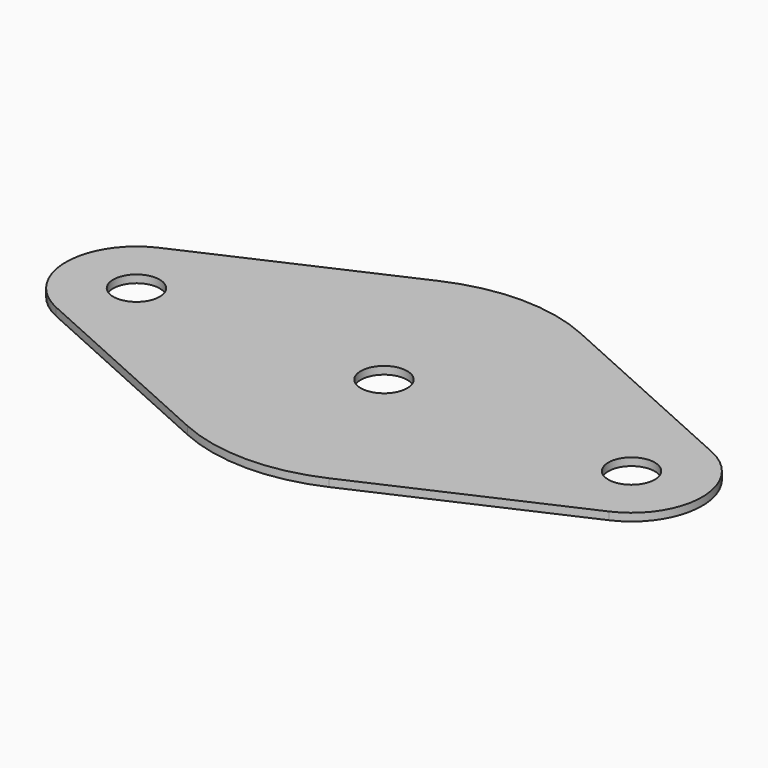
from build123d import *

# Parameters (mm, degrees)
F0_R     = 13.9065
F0_R_2   = 9.525
F1_DEPTH = 3.175


# Not quite as in the source:
# - a length typed as a fraction of an inch, garbled in the dataset ("3 / 203.2 mm" for 3/8 in), is restored


with BuildPart() as f1:
    # F0 (on Top) → F1 (new body)
    with BuildSketch(Plane.XY):
        with BuildLine():
            Line((70.7064372, 0), (64.77, 0))
            ThreePointArc((64.77, 0), (0, -64.77), (-64.77, 0))
            Line((-64.77, 0), (-70.7064372, 0))
            ThreePointArc((-70.7064372, 0), (-59.3851891605, -38.3770708873), (-29.0468761129, -64.4645580889))
            ThreePointArc((-29.0468761129, -64.4645580889), (0, -70.7064372), (29.0468761129, -64.4645580889))
            ThreePointArc((29.0468761129, -64.4645580889), (59.3851891605, -38.3770708873), (70.7064372, 0))
        make_face()
        with BuildLine():
            ThreePointArc((-64.77, 0), (0, 64.77), (64.77, 0))
            Line((64.77, 0), (70.7064372, 0))
            ThreePointArc((70.7064372, 0), (59.3851891605, 38.3770708873), (29.0468761129, 64.4645580889))
            ThreePointArc((29.0468761129, 64.4645580889), (0, 70.7064372), (-29.0468761129, 64.4645580889))
            ThreePointArc((-29.0468761129, 64.4645580889), (-59.3851891605, 38.3770708873), (-70.7064372, 0))
            Line((-70.7064372, 0), (-64.77, 0))
        make_face()
        with BuildLine():
            Line((72.631808, 0), (70.7064372, 0))
            ThreePointArc((70.7064372, 0), (59.3851891605, -38.3770708873), (29.0468761129, -64.4645580889))
            Line((29.0468761129, -64.4645580889), (113.5004084714, -26.410914902))
            ThreePointArc((113.5004084714, -26.410914902), (85.8770417817, -24.3299143569), (72.631808, 0))
        make_face()
        with BuildLine():
            ThreePointArc((29.0468761129, 64.4645580889), (59.3851891605, 38.3770708873), (70.7064372, 0))
            Line((70.7064372, 0), (72.631808, 0))
            ThreePointArc((72.631808, 0), (85.8770417817, 24.3299143569), (113.5004084714, 26.410914902))
            Line((113.5004084714, 26.410914902), (29.0468761129, 64.4645580889))
        make_face()
        with BuildLine():
            Line((-72.631808, 0), (-70.7064372, 0))
            ThreePointArc((-70.7064372, 0), (-59.3851891605, 38.3770708873), (-29.0468761129, 64.4645580889))
            Line((-29.0468761129, 64.4645580889), (-113.5004084714, 26.410914902))
            ThreePointArc((-113.5004084714, 26.410914902), (-85.8770417817, 24.3299143569), (-72.631808, 0))
        make_face()
        with BuildLine():
            ThreePointArc((-29.0468761129, -64.4645580889), (-59.3851891605, -38.3770708873), (-70.7064372, 0))
            Line((-70.7064372, 0), (-72.631808, 0))
            ThreePointArc((-72.631808, 0), (-85.8770417817, -24.3299143569), (-113.5004084714, -26.410914902))
            Line((-113.5004084714, -26.410914902), (-29.0468761129, -64.4645580889))
        make_face()
        with BuildLine():
            ThreePointArc((113.5004084714, 26.410914902), (85.8770417817, 24.3299143569), (72.631808, 0))
            ThreePointArc((72.631808, 0), (85.8770417817, -24.3299143569), (113.5004084714, -26.410914902))
            ThreePointArc((113.5004084714, -26.410914902), (125.9299143569, -15.7229582183), (130.568192, 0))
            ThreePointArc((130.568192, 0), (125.9299143569, 15.7229582183), (113.5004084714, 26.410914902))
        make_face()
        with BuildLine():
            ThreePointArc((115.5065, 0), (101.6, -13.9065), (87.6935, 0))
            ThreePointArc((87.6935, 0), (101.6, 13.9065), (115.5065, 0))
        make_face(mode=Mode.SUBTRACT)
        with BuildLine():
            ThreePointArc((-113.5004084714, -26.410914902), (-85.8770417817, -24.3299143569), (-72.631808, 0))
            ThreePointArc((-72.631808, 0), (-85.8770417817, 24.3299143569), (-113.5004084714, 26.410914902))
            ThreePointArc((-113.5004084714, 26.410914902), (-130.568192, 0), (-113.5004084714, -26.410914902))
        make_face()
        with Locations((-101.6, 0)):
            Circle(F0_R, mode=Mode.SUBTRACT)
        with BuildLine():
            ThreePointArc((-64.77, 0), (0, -64.77), (64.77, 0))
            Line((64.77, 0), (9.525, 0))
            ThreePointArc((9.525, 0), (0, -9.525), (-9.525, 0))
            Line((-9.525, 0), (-64.77, 0))
        make_face()
        with BuildLine():
            Line((9.525, 0), (64.77, 0))
            ThreePointArc((64.77, 0), (0, 64.77), (-64.77, 0))
            Line((-64.77, 0), (-9.525, 0))
            ThreePointArc((-9.525, 0), (0, 9.525), (9.525, 0))
        make_face()
        with BuildLine():
            ThreePointArc((115.5065, 0), (101.6, 13.9065), (87.6935, 0))
            ThreePointArc((87.6935, 0), (101.6, -13.9065), (115.5065, 0))
        make_face()
        with BuildLine():
            ThreePointArc((111.125, 0), (101.6, -9.525), (92.075, 0))
            ThreePointArc((92.075, 0), (101.6, 9.525), (111.125, 0))
        make_face(mode=Mode.SUBTRACT)
        with Locations((-101.6, 0)):
            Circle(F0_R)
        with Locations((-101.6, 0)):
            Circle(F0_R_2, mode=Mode.SUBTRACT)
    extrude(amount=F1_DEPTH)


solid = f1.part
